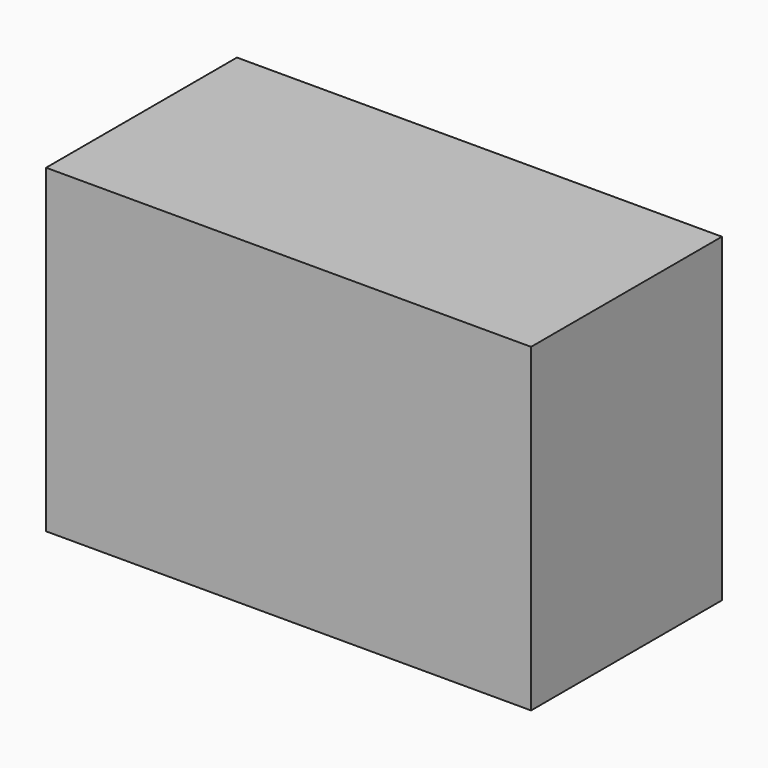
from build123d import *

# Parameters (mm, degrees)
F0_W     = 51.6358476598
F0_H     = 34.0830702335
F1_DEPTH = 25.4


# Not quite as in the source:
# - the program builds the solid bodies; features that only make, move or delete a surface that nothing else refers to are left out


with BuildPart() as f1:
    # F0 (on Front) → F1 (new body)
    with BuildSketch(Plane.XZ):
        with Locations((-28.3741535386, 37.0653374121)):
            Rectangle(F0_W, F0_H)
    extrude(amount=F1_DEPTH)


with BuildPart() as f1b:
    # F0 (on Front) → F1, piece 2 (new body)
    with BuildSketch(Plane.XZ):
        with BuildLine():
            add(Edge.make_bspline(
                [(22.3244093359, -13.7184355408), (20.9649784334, -4.7843207272), (25.9798632943, 15.3706872491), (65.2765981799, 46.8827002107), (65.9557933658, 4.9138085279), (31.1793653474, -36.4502806513), (23.2965008124, -20.1069741898), (22.3244093359, -13.7184355408)],
                knots=[0, 0, 0, 0, 0.2008979891, 0.4184498703, 0.6092802876, 0.8563433989, 1, 1, 1, 1], degree=3))
        make_face()
    extrude(amount=F1_DEPTH)


solid = f1.part
